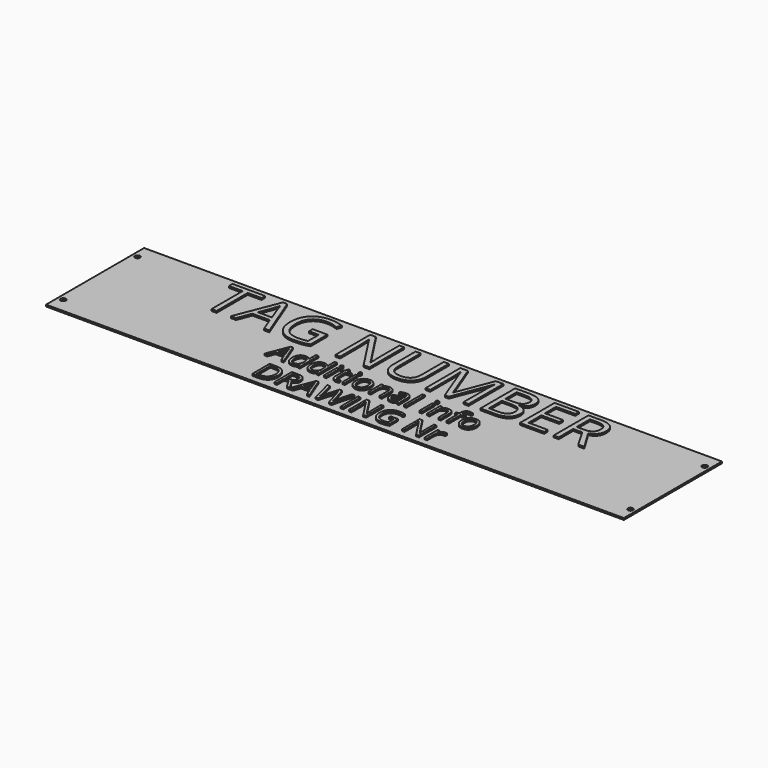
from build123d import *

# Parameters (mm, degrees)
F0_W           = 330
F0_H           = 70
F0_R           = 1.5
F1_DEPTH       = 1
F2_TEXT_SIZE   = 34.7361111111
F2_TEXT_SIZE_2 = 17.3611111111
F3_DEPTH       = 1


# Not quite as in the source:
# - Text() gives the source's letters only with a copy of the font that has no kerning and outlines rounded to 1/6400 em; it was checked with that copy


with BuildPart() as f1:
    # F0 (on Top) → F1 (new body)
    with BuildSketch(Plane.XY):
        Rectangle(F0_W, F0_H)
        with Locations((-162, -26.5)):
            Circle(F0_R, mode=Mode.SUBTRACT)
        with Locations((162, -26.5)):
            Circle(F0_R, mode=Mode.SUBTRACT)
        with Locations((-162, 26.5)):
            Circle(F0_R, mode=Mode.SUBTRACT)
        with Locations((162, 26.5)):
            Circle(F0_R, mode=Mode.SUBTRACT)
    extrude(amount=F1_DEPTH)


with BuildPart() as f3:
    # F2 (on face) → F3 (new body)
    with BuildSketch(Plane.XY.offset(1)):
        with Locations((-111.6521733941, 6.245)):
            Text('TAG NUMBER', F2_TEXT_SIZE, font='Open Sans', text_align=(TextAlign.LEFT, TextAlign.BOTTOM))
        with Locations((-51.8931865545, -31.255)):
            Text('DRAWING Nr', F2_TEXT_SIZE_2, font='Open Sans', text_align=(TextAlign.LEFT, TextAlign.BOTTOM))
        with Locations((-58.1150093257, -12.505)):
            Text('Additional info', F2_TEXT_SIZE_2, font='Open Sans', text_align=(TextAlign.LEFT, TextAlign.BOTTOM))
    extrude(amount=F3_DEPTH)


solid = Compound([f1.part, f3.part])
